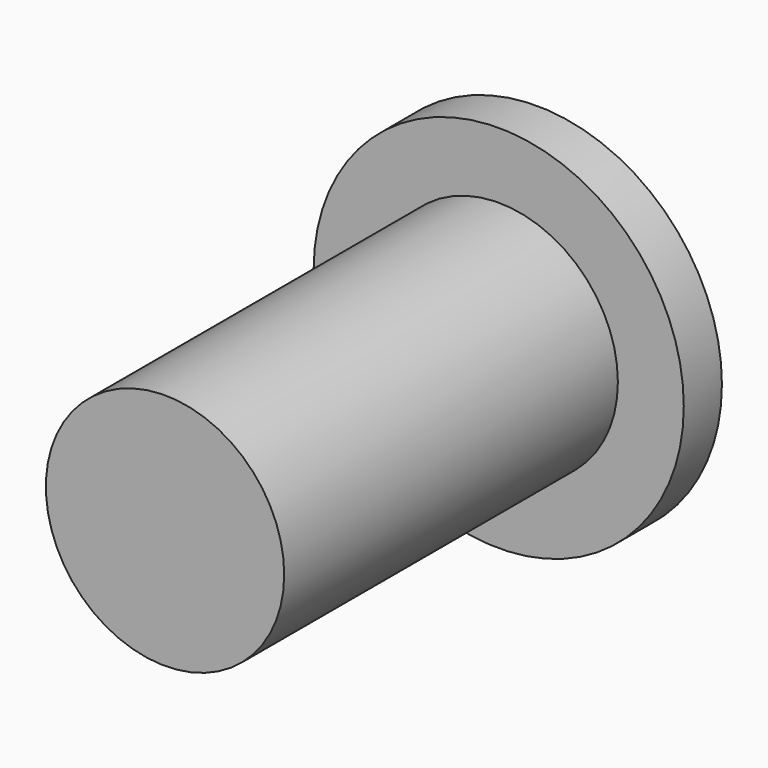
from build123d import *

# Parameters (mm, degrees)
F0_R     = 20
F1_DEPTH = 70
F2_R     = 31.0612290884
F2_R_2   = 20
F3_DEPTH = 8


with BuildPart() as f1:
    # F0 (on Front) → F1 (new body)
    with BuildSketch(Plane.XZ):
        Circle(F0_R)
    extrude(amount=F1_DEPTH)

    # F2 (on face) → F3 (join)
    with BuildSketch(Plane(origin=(0, 0, 0), x_dir=(-1, 0, 0), z_dir=(0, 1, 0))):
        Circle(F2_R)
        Circle(F2_R_2, mode=Mode.SUBTRACT)
        Circle(F2_R_2)
    extrude(amount=F3_DEPTH)


solid = f1.part
